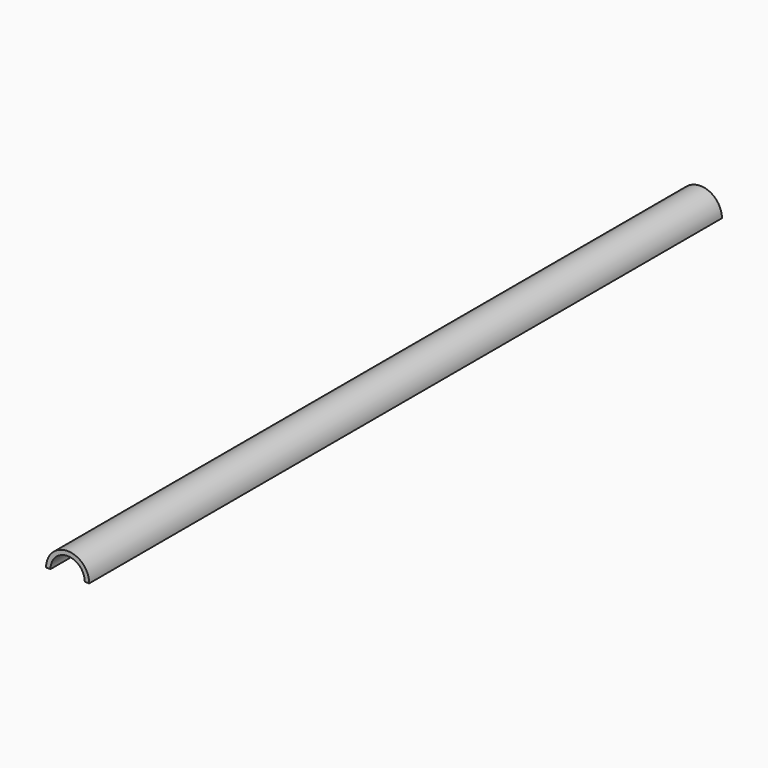
from build123d import *

# Parameters (mm, degrees)
F1_DEPTH = 1000


# Not quite as in the source:
# - the program builds the solid bodies; features that only make, move or delete a surface that nothing else refers to are left out


with BuildPart() as f1:
    # F0 (on Front) → F1 (new body)
    with BuildSketch(Plane.XZ):
        with BuildLine():
            ThreePointArc((-21.6923840344, 0), (0, 21.6923840344), (21.6923840344, 0))
            Line((21.6923840344, 0), (27.2473022342, 0))
            ThreePointArc((27.2473022342, 0), (0, 27.2473022342), (-27.2473022342, 0))
            Line((-27.2473022342, 0), (-21.6923840344, 0))
        make_face()
    extrude(amount=F1_DEPTH)


solid = f1.part
